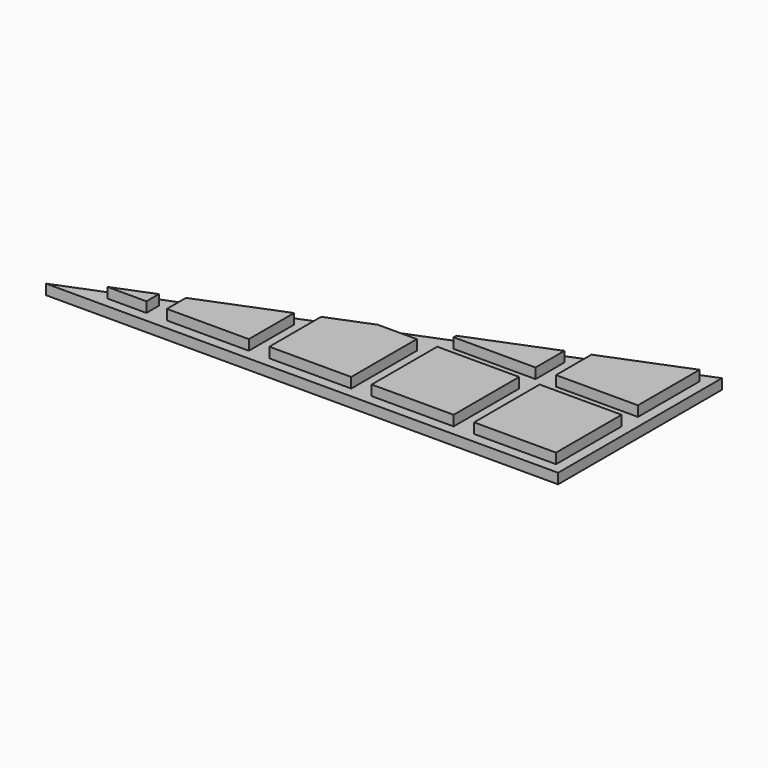
from build123d import *

# Parameters (mm, degrees)
F1_DEPTH = 1
F2_W     = 8
F2_H     = 8
F3_DEPTH = 1


# Not quite as in the source:
# - a feature names something its author has since deleted; it is built from what else it names


with BuildPart() as f1:
    # F0 (on Top) → F1 (new body)
    with BuildSketch(Plane.XY):
        Polygon((0, 20), (-50, 0), (0, 0), align=None)
    extrude(amount=F1_DEPTH)

    # F2 (on face) → F3 (join)
    with BuildSketch(Plane.XY.offset(1)):
        Polygon((-19, 11.3229670386), (-19, 11), (-11, 11), (-11, 14.5229670386), align=None)
        Polygon((-29, 7.3229670386), (-29, 1), (-21, 1), (-21, 9), (-24.8074175964, 9), align=None)
        Polygon((-39, 3.3229670386), (-39, 1), (-31, 1), (-31, 6.5229670386), align=None)
        Polygon((-9, 15.3229670386), (-9, 11), (-1, 11), (-1, 18.5229670386), align=None)
        with Locations((-5, 5)):
            Rectangle(F2_W, F2_H)
        with Locations((-15, 5)):
            Rectangle(F2_W, F2_H)
        Polygon((-41, 2.5229670386), (-44.8074175964, 1), (-41, 1), align=None)
    extrude(amount=F3_DEPTH)


solid = f1.part
